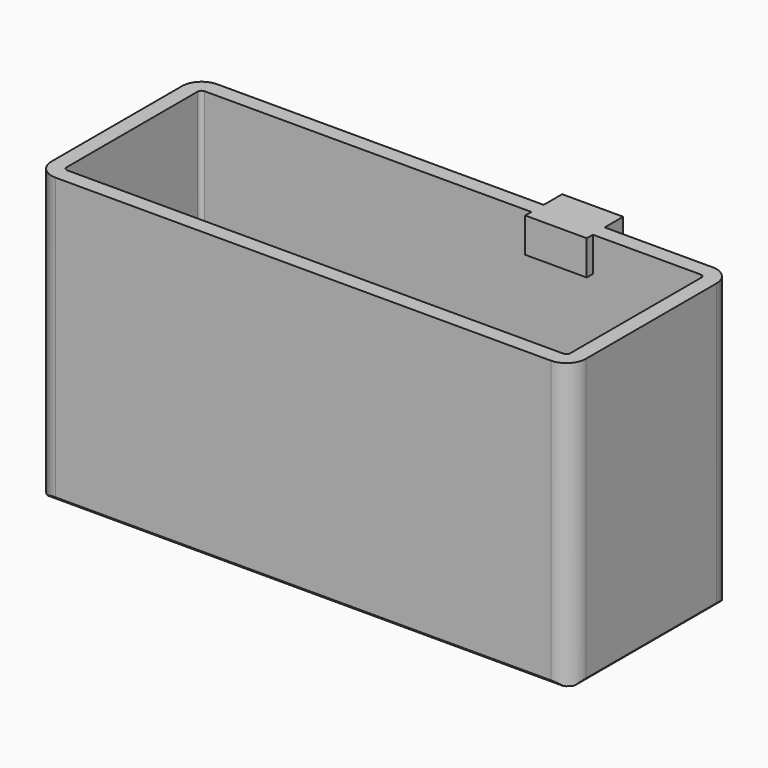
from build123d import *

# Parameters (mm, degrees)
F0_W        = 69.5
F0_H        = 26.3
F1_DEPTH    = 37
F2_W        = 65.5
F2_H        = 22.3
F3_DEPTH    = 35
F4_SIZE     = 0.4
F5_T1_DEPTH = 49.3
F6_R        = 2.54
F7_W        = 8
F7_H        = 4.5
F8_DEPTH    = 1
F9_W        = 7.9342592508
F9_H        = 2.0083109736
F10_DEPTH   = 3
F11_R       = 0.5


# Not quite as in the source:
# - a fillet or chamfer that OpenCascade refuses, or shapes differently, is made with other operations: its cross-section is extruded or revolved along the edge and cut away or added


with BuildPart() as f1:
    # F0 (on Top) → F1 (new body)
    with BuildSketch(Plane.XY):
        Rectangle(F0_W, F0_H)
    extrude(amount=F1_DEPTH)

    # F2 (on face) → F3 (cut)
    with BuildSketch(Plane.XY.offset(37)):
        Rectangle(F2_W, F2_H)
    extrude(amount=-F3_DEPTH, mode=Mode.SUBTRACT)

    # F4
    f4_edges = [f1.edges().sort_by_distance(p)[0] for p in [
        (0, -13.15, 0),
        (34.75, 0, 0),
        (0, 13.15, 0),
        (-34.75, 0, 0),
    ]]
    chamfer(f4_edges, length=F4_SIZE)

    # F5: fillet of radius 2.54 on 4 edges, made by hand

    # F5_s2 → F5_t1 (cut)
    with BuildSketch(Plane.XY.offset(-5.95)):
        with BuildLine():
            ThreePointArc((34.75, 10.61), (34.0060512242, 12.4060512242), (32.21, 13.15))
            Line((32.21, 13.15), (34.75, 13.15))
            Line((34.75, 13.15), (34.75, 10.61))
        make_face()
        with BuildLine():
            ThreePointArc((32.21, -13.15), (34.0060512242, -12.4060512242), (34.75, -10.61))
            Line((34.75, -10.61), (34.75, -13.15))
            Line((34.75, -13.15), (32.21, -13.15))
        make_face()
        with BuildLine():
            ThreePointArc((-34.75, 10.61), (-34.0060512242, 12.4060512242), (-32.21, 13.15))
            Line((-32.21, 13.15), (-34.75, 13.15))
            Line((-34.75, 13.15), (-34.75, 10.61))
        make_face()
        with BuildLine():
            ThreePointArc((-32.21, -13.15), (-34.0060512242, -12.4060512242), (-34.75, -10.61))
            Line((-34.75, -10.61), (-34.75, -13.15))
            Line((-34.75, -13.15), (-32.21, -13.15))
        make_face()
    extrude(amount=F5_T1_DEPTH, mode=Mode.SUBTRACT)

    # F6
    f6_edges = [f1.edges().sort_by_distance(p)[0] for p in [
        (0, -11.15, 2),
        (-32.75, 0, 2),
        (32.75, 0, 2),
        (0, 11.15, 2),
    ]]
    fillet(f6_edges, radius=F6_R)

    # F7 (on face) → F8 (join)
    with BuildSketch(Plane.XZ.offset(-11.15)):
        with Locations((14.25, 34.75)):
            Rectangle(F7_W, F7_H)
    extrude(amount=F8_DEPTH)

    # F9 (on face) → F10 (join)
    with BuildSketch(Plane(origin=(0, 13.15, 0), x_dir=(-1, 0, 0), z_dir=(0, 1, 0))):
        with Locations((-14.2189497128, 35.9958445132)):
            Rectangle(F9_W, F9_H)
    extrude(amount=F10_DEPTH)

    # F11
    f11_edges = [f1.edges().sort_by_distance(p)[0] for p in [
        (32.75, 11.15, 20.77),
        (32.75, -11.15, 20.77),
        (-32.75, -11.15, 20.77),
        (-32.75, 11.15, 20.77),
    ]]
    fillet(f11_edges, radius=F11_R)


solid = f1.part
